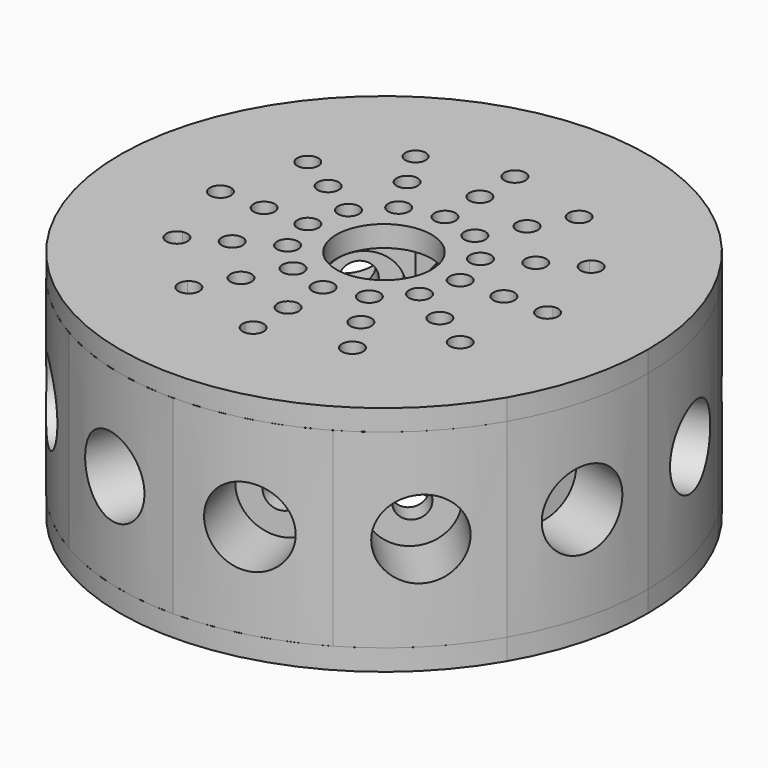
from build123d import *
from build123d import SkipClean  # not in build123d's __all__

# Parameters (mm, degrees)
F1_DEPTH  = 18
F2_R      = 3.35
F2_R_2    = 1.5
F3_DEPTH  = 2
F4_DEPTH  = 12
F6_R      = 3.7
F7_DEPTH  = 12
F8_R      = 1
F9_DEPTH  = 2
F10_R     = 1
F11_DEPTH = 2
F12_COUNT = 12
F13_R     = 1
F13_R_2   = 0.75
F13_R_3   = 4.5
F14_DEPTH = 2
F15_DEPTH = 1.5
F16_R     = 1
F16_R_2   = 1.0601015706
F16_R_3   = 4.5
F16_R_4   = 0.75
F17_DEPTH = 2
F18_DEPTH = 1.5


with BuildPart() as f1:
    # F0 (on Top) → F1 (new body)
    with BuildSketch(Plane.XY):
        with BuildLine():
            Line((7.75, 13.4233937587), (12.5, 21.6506350946))
            ThreePointArc((12.5, 21.6506350946), (6.4704761276, 24.1481456572), (0, 25))
            Line((0, 25), (0, 15.5))
            Line((0, 15.5), (7.75, 13.4233937587))
        make_face()
    extrude(amount=F1_DEPTH)

    # F2 (on face) → F3 (cut)
    with BuildSketch(Plane(origin=(3.875, 14.4616968793, 0), x_dir=(0.9659258263, -0.2588190451, 0), z_dir=(-0.2588190451, -0.9659258263, 0))):
        with Locations((0, 9)):
            Circle(F2_R)
        with Locations((0, 9)):
            Circle(F2_R_2, mode=Mode.SUBTRACT)
    extrude(amount=-F3_DEPTH, mode=Mode.SUBTRACT)

    # F4 (cut): a face of the model
    f4_faces = [f1.faces().sort_by_distance(p)[0] for p in [
        (3.875, 14.4616968793, 9),
    ]]
    extrude(f4_faces, amount=-F4_DEPTH, mode=Mode.SUBTRACT)

    # F6 (on offset) → F7 (cut)
    with BuildSketch(Plane(origin=(4.9102761804, 18.3254001845, 0), x_dir=(0.9659258263, -0.2588190451, 0), z_dir=(-0.2588190451, -0.9659258263, 0))):
        with Locations((0, 9)):
            Circle(F6_R)
    extrude(amount=-F7_DEPTH, mode=Mode.SUBTRACT)

    # F8 (on face) → F9 (cut)
    with BuildSketch(Plane.XY.offset(18)):
        with Locations((9.7439876188, 20.8650568617)):
            Circle(F8_R)
    extrude(amount=-F9_DEPTH, mode=Mode.SUBTRACT)

    # F10 (on face) → F11 (cut)
    with BuildSketch(Plane(origin=(0, 0, 0), x_dir=(1, 0, 0), z_dir=(0, 0, -1))):
        with Locations((1.9939876188, -22.941663103)):
            Circle(F10_R)
    extrude(amount=-F11_DEPTH, mode=Mode.SUBTRACT)

    # F12: F1 ×12 about axis
    f12_axis = Axis((0, 0, 0), (0, 0, 1))


with BuildPart() as f1_1:
    add(f1.part, clean=False)
    with SkipClean():  # cleaning this boolean's faces spoils the solid; the shape is the same uncleaned
        for i in range(1, F12_COUNT):
            add(f1.part.rotate(f12_axis, i * 360 / F12_COUNT), clean=False)


with BuildPart() as f14:
    # F13 (on face) → F14 (new body)
    with BuildSketch(Plane.XY.offset(18)):
        with BuildLine():
            Line((14.2894191624, 8.25), (21.6506350946, 12.5))
            ThreePointArc((21.6506350946, 12.5), (17.6776695297, 17.6776695297), (12.5, 21.6506350946))
            Line((12.5, 21.6506350946), (8.25, 14.2894191624))
            ThreePointArc((8.25, 14.2894191624), (8.6160254038, 13.9233937587), (8.75, 13.4233937587))
            ThreePointArc((8.75, 13.4233937587), (8.6738795325, 13.0407103263), (8.4571067812, 12.7162869775))
            Line((8.4571067812, 12.7162869775), (12.7162869775, 8.4571067812))
            ThreePointArc((12.7162869775, 8.4571067812), (13.5539199509, 8.7414448614), (14.2894191624, 8.25))
        make_face()
        with Locations((18.8710692429, 13.1976754842)):
            Circle(F13_R, mode=Mode.SUBTRACT)
        with BuildLine():
            ThreePointArc((21.6506350946, -12.5), (24.1481456572, -6.4704761276), (25, 0))
            ThreePointArc((25, 0), (24.1481456572, 6.4704761276), (21.6506350946, 12.5))
            Line((21.6506350946, 12.5), (14.2894191624, 8.25))
            ThreePointArc((14.2894191624, 8.25), (14.3893195849, 8.0088190451), (14.4233937587, 7.75))
            ThreePointArc((14.4233937587, 7.75), (14.216747099, 7.141238571), (13.6822128038, 6.7840741737))
            Line((13.6822128038, 6.7840741737), (15.2411809549, 0.9659258263))
            ThreePointArc((15.2411809549, 0.9659258263), (16.108761429, 0.7933533403), (16.5, 0))
            ThreePointArc((16.5, 0), (16.108761429, -0.7933533403), (15.2411809549, -0.9659258263))
            Line((15.2411809549, -0.9659258263), (13.6822128038, -6.7840741737))
            ThreePointArc((13.6822128038, -6.7840741737), (14.216747099, -7.141238571), (14.4233937587, -7.75))
            ThreePointArc((14.4233937587, -7.75), (13.806077191, -8.6738795325), (12.7162869775, -8.4571067812))
            Line((12.7162869775, -8.4571067812), (8.4571067812, -12.7162869775))
            ThreePointArc((8.4571067812, -12.7162869775), (8.6738795325, -13.0407103263), (8.75, -13.4233937587))
            ThreePointArc((8.75, -13.4233937587), (7.8805261922, -14.41483862), (6.7840741737, -13.6822128038))
            Line((6.7840741737, -13.6822128038), (0.9659258263, -15.2411809549))
            ThreePointArc((0.9659258263, -15.2411809549), (0.9914448614, -15.3694738078), (1, -15.5))
            ThreePointArc((1, -15.5), (-0.1305261922, -16.4914448614), (-0.9659258263, -15.2411809549))
            Line((-0.9659258263, -15.2411809549), (-6.7840741737, -13.6822128038))
            ThreePointArc((-6.7840741737, -13.6822128038), (-8.25, -14.2894191624), (-8.4571067812, -12.7162869775))
            Line((-8.4571067812, -12.7162869775), (-12.7162869775, -8.4571067812))
            ThreePointArc((-12.7162869775, -8.4571067812), (-14.2894191624, -8.25), (-13.6822128038, -6.7840741737))
            Line((-13.6822128038, -6.7840741737), (-15.2411809549, -0.9659258263))
            ThreePointArc((-15.2411809549, -0.9659258263), (-16.5, 0), (-15.2411809549, 0.9659258263))
            Line((-15.2411809549, 0.9659258263), (-13.6822128038, 6.7840741737))
            ThreePointArc((-13.6822128038, 6.7840741737), (-14.2894191624, 8.25), (-12.7162869775, 8.4571067812))
            Line((-12.7162869775, 8.4571067812), (-8.4328611299, 12.7405326287))
            ThreePointArc((-8.4328611299, 12.7405326287), (-8.2328557356, 14.2597244254), (-6.8171943493, 13.6733382795))
            Line((-6.8171943493, 13.6733382795), (-0.9659258263, 15.2411809549))
            ThreePointArc((-0.9659258263, 15.2411809549), (-0.1305261922, 16.4914448614), (1, 15.5))
            ThreePointArc((1, 15.5), (0.9914448614, 15.3694738078), (0.9659258263, 15.2411809549))
            Line((0.9659258263, 15.2411809549), (6.7840741737, 13.6822128038))
            ThreePointArc((6.7840741737, 13.6822128038), (7.3673165676, 14.3472732912), (8.25, 14.2894191624))
            Line((8.25, 14.2894191624), (12.5, 21.6506350946))
            ThreePointArc((12.5, 21.6506350946), (-24.1481456572, -6.4704761276), (21.6506350946, -12.5))
        make_face()
        with Locations((-18.8710692429, -13.1976754842)):
            Circle(F13_R, mode=Mode.SUBTRACT)
        with Locations((-9.7439876188, -20.8650568617)):
            Circle(F13_R, mode=Mode.SUBTRACT)
        with Locations((-22.941663103, -1.9939876188)):
            Circle(F13_R, mode=Mode.SUBTRACT)
        with Locations((1.9939876188, -22.941663103)):
            Circle(F13_R, mode=Mode.SUBTRACT)
        with Locations((13.1976754842, -18.8710692429)):
            Circle(F13_R, mode=Mode.SUBTRACT)
        with Locations((20.8650568617, -9.7439876188)):
            Circle(F13_R, mode=Mode.SUBTRACT)
        with Locations((-20.8650568617, 9.7439876188)):
            Circle(F13_R, mode=Mode.SUBTRACT)
        with Locations((-13.1976754842, 18.8710692429)):
            Circle(F13_R, mode=Mode.SUBTRACT)
        with Locations((-1.9939876188, 22.941663103)):
            Circle(F13_R, mode=Mode.SUBTRACT)
        with Locations((22.941663103, 1.9939876188)):
            Circle(F13_R, mode=Mode.SUBTRACT)
        with Locations((9.7439876188, 20.8650568617)):
            Circle(F13_R, mode=Mode.SUBTRACT)
        with Locations((-20.8650568617, 9.7439876188)):
            Circle(F13_R)
        with Locations((-20.8650568617, 9.7439876188)):
            Circle(F13_R_2, mode=Mode.SUBTRACT)
        with Locations((-22.941663103, -1.9939876188)):
            Circle(F13_R)
        with Locations((-22.941663103, -1.9939876188)):
            Circle(F13_R_2, mode=Mode.SUBTRACT)
        with BuildLine():
            ThreePointArc((13.6822128038, 6.7840741737), (12.5573683549, 7.25), (12.7162869775, 8.4571067812))
            Line((12.7162869775, 8.4571067812), (8.4571067812, 12.7162869775))
            ThreePointArc((8.4571067812, 12.7162869775), (7.25, 12.5573683549), (6.7840741737, 13.6822128038))
            Line((6.7840741737, 13.6822128038), (0.9659258263, 15.2411809549))
            ThreePointArc((0.9659258263, 15.2411809549), (0, 14.5), (-0.9659258263, 15.2411809549))
            Line((-0.9659258263, 15.2411809549), (-6.8171943493, 13.6733382795))
            ThreePointArc((-6.8171943493, 13.6733382795), (-6.7925503244, 13.5494443998), (-6.7842885289, 13.4233937587))
            ThreePointArc((-6.7842885289, 13.4233937587), (-7.3804382195, 12.5311926962), (-8.4328611299, 12.7405326287))
            Line((-8.4328611299, 12.7405326287), (-12.7162869775, 8.4571067812))
            ThreePointArc((-12.7162869775, 8.4571067812), (-12.4995142261, 8.1326834324), (-12.4233937587, 7.75))
            ThreePointArc((-12.4233937587, 7.75), (-12.8146323297, 6.9566466597), (-13.6822128038, 6.7840741737))
            Line((-13.6822128038, 6.7840741737), (-15.2411809549, 0.9659258263))
            ThreePointArc((-15.2411809549, 0.9659258263), (-14.7066466597, 0.608761429), (-14.5, 0))
            ThreePointArc((-14.5, 0), (-14.7066466597, -0.608761429), (-15.2411809549, -0.9659258263))
            Line((-15.2411809549, -0.9659258263), (-13.6822128038, -6.7840741737))
            ThreePointArc((-13.6822128038, -6.7840741737), (-12.8146323297, -6.9566466597), (-12.4233937587, -7.75))
            ThreePointArc((-12.4233937587, -7.75), (-12.4995142261, -8.1326834324), (-12.7162869775, -8.4571067812))
            Line((-12.7162869775, -8.4571067812), (-8.4571067812, -12.7162869775))
            ThreePointArc((-8.4571067812, -12.7162869775), (-7.3673165676, -12.4995142261), (-6.75, -13.4233937587))
            ThreePointArc((-6.75, -13.4233937587), (-6.7585551386, -13.5539199509), (-6.7840741737, -13.6822128038))
            Line((-6.7840741737, -13.6822128038), (-0.9659258263, -15.2411809549))
            ThreePointArc((-0.9659258263, -15.2411809549), (0, -14.5), (0.9659258263, -15.2411809549))
            Line((0.9659258263, -15.2411809549), (6.7840741737, -13.6822128038))
            ThreePointArc((6.7840741737, -13.6822128038), (7.25, -12.5573683549), (8.4571067812, -12.7162869775))
            Line((8.4571067812, -12.7162869775), (12.7162869775, -8.4571067812))
            ThreePointArc((12.7162869775, -8.4571067812), (12.5573683549, -7.25), (13.6822128038, -6.7840741737))
            Line((13.6822128038, -6.7840741737), (15.2411809549, -0.9659258263))
            ThreePointArc((15.2411809549, -0.9659258263), (14.5, 0), (15.2411809549, 0.9659258263))
            Line((15.2411809549, 0.9659258263), (13.6822128038, 6.7840741737))
        make_face()
        with Locations((-5.6794476392, -9.83709187)):
            Circle(F13_R, mode=Mode.SUBTRACT)
        with Locations((-3.6088952784, -6.2507899813)):
            Circle(F13_R, mode=Mode.SUBTRACT)
        with Locations((-9.83709187, -5.6794476392)):
            Circle(F13_R, mode=Mode.SUBTRACT)
        with Locations((-6.2507899813, -3.6088952784)):
            Circle(F13_R, mode=Mode.SUBTRACT)
        with Locations((0, -11.3588952784)):
            Circle(F13_R, mode=Mode.SUBTRACT)
        with Locations((5.6794476392, -9.83709187)):
            Circle(F13_R, mode=Mode.SUBTRACT)
        with Locations((0, -7.2177905567)):
            Circle(F13_R, mode=Mode.SUBTRACT)
        with Locations((3.6088952784, -6.2507899813)):
            Circle(F13_R, mode=Mode.SUBTRACT)
        with Locations((6.2507899813, -3.6088952784)):
            Circle(F13_R, mode=Mode.SUBTRACT)
        with Locations((9.83709187, -5.6794476392)):
            Circle(F13_R, mode=Mode.SUBTRACT)
        with Locations((-11.3588952784, 0)):
            Circle(F13_R, mode=Mode.SUBTRACT)
        with Locations((-7.2177905567, 0)):
            Circle(F13_R, mode=Mode.SUBTRACT)
        with Locations((-9.83709187, 5.6794476392)):
            Circle(F13_R, mode=Mode.SUBTRACT)
        with Locations((-6.2507899813, 3.6088952784)):
            Circle(F13_R, mode=Mode.SUBTRACT)
        with Locations((-3.6088952784, 6.2507899813)):
            Circle(F13_R, mode=Mode.SUBTRACT)
        with Locations((-5.6794476392, 9.83709187)):
            Circle(F13_R, mode=Mode.SUBTRACT)
        Circle(F13_R_3, mode=Mode.SUBTRACT)
        with Locations((7.2177905567, 0)):
            Circle(F13_R, mode=Mode.SUBTRACT)
        with Locations((11.3588952784, 0)):
            Circle(F13_R, mode=Mode.SUBTRACT)
        with Locations((6.2507899813, 3.6088952784)):
            Circle(F13_R, mode=Mode.SUBTRACT)
        with Locations((9.83709187, 5.6794476392)):
            Circle(F13_R, mode=Mode.SUBTRACT)
        with Locations((0, 7.2177905567)):
            Circle(F13_R, mode=Mode.SUBTRACT)
        with Locations((3.6088952784, 6.2507899813)):
            Circle(F13_R, mode=Mode.SUBTRACT)
        with Locations((0, 11.3588952784)):
            Circle(F13_R, mode=Mode.SUBTRACT)
        with Locations((5.6794476392, 9.83709187)):
            Circle(F13_R, mode=Mode.SUBTRACT)
        with Locations((-18.8710692429, -13.1976754842)):
            Circle(F13_R)
        with Locations((-18.8710692429, -13.1976754842)):
            Circle(F13_R_2, mode=Mode.SUBTRACT)
        with Locations((-9.7439876188, -20.8650568617)):
            Circle(F13_R)
        with Locations((-9.7439876188, -20.8650568617)):
            Circle(F13_R_2, mode=Mode.SUBTRACT)
        with Locations((1.9939876188, -22.941663103)):
            Circle(F13_R)
        with Locations((1.9939876188, -22.941663103)):
            Circle(F13_R_2, mode=Mode.SUBTRACT)
        with Locations((13.1976754842, -18.8710692429)):
            Circle(F13_R)
        with Locations((13.1976754842, -18.8710692429)):
            Circle(F13_R_2, mode=Mode.SUBTRACT)
        with Locations((20.8650568617, -9.7439876188)):
            Circle(F13_R)
        with Locations((20.8650568617, -9.7439876188)):
            Circle(F13_R_2, mode=Mode.SUBTRACT)
        with Locations((22.941663103, 1.9939876188)):
            Circle(F13_R)
        with Locations((22.941663103, 1.9939876188)):
            Circle(F13_R_2, mode=Mode.SUBTRACT)
        with Locations((18.8710692429, 13.1976754842)):
            Circle(F13_R)
        with Locations((18.8710692429, 13.1976754842)):
            Circle(F13_R_2, mode=Mode.SUBTRACT)
        with Locations((9.7439876188, 20.8650568617)):
            Circle(F13_R)
        with Locations((9.7439876188, 20.8650568617)):
            Circle(F13_R_2, mode=Mode.SUBTRACT)
        with Locations((-1.9939876188, 22.941663103)):
            Circle(F13_R)
        with Locations((-1.9939876188, 22.941663103)):
            Circle(F13_R_2, mode=Mode.SUBTRACT)
        with Locations((-13.1976754842, 18.8710692429)):
            Circle(F13_R)
        with Locations((-13.1976754842, 18.8710692429)):
            Circle(F13_R_2, mode=Mode.SUBTRACT)
        with Locations((-22.941663103, -1.9939876188)):
            Circle(F13_R_2)
        with Locations((-20.8650568617, 9.7439876188)):
            Circle(F13_R_2)
        with Locations((-18.8710692429, -13.1976754842)):
            Circle(F13_R_2)
        with Locations((20.8650568617, -9.7439876188)):
            Circle(F13_R_2)
        with Locations((22.941663103, 1.9939876188)):
            Circle(F13_R_2)
        with Locations((18.8710692429, 13.1976754842)):
            Circle(F13_R_2)
        with Locations((-9.7439876188, -20.8650568617)):
            Circle(F13_R_2)
        with Locations((1.9939876188, -22.941663103)):
            Circle(F13_R_2)
        with Locations((13.1976754842, -18.8710692429)):
            Circle(F13_R_2)
        with Locations((-1.9939876188, 22.941663103)):
            Circle(F13_R_2)
        with Locations((9.7439876188, 20.8650568617)):
            Circle(F13_R_2)
        with Locations((-13.1976754842, 18.8710692429)):
            Circle(F13_R_2)
    extrude(amount=F14_DEPTH)

    # F13 (on face) → F15 (join)
    with BuildSketch(Plane.XY.offset(18)):
        with Locations((-13.1976754842, 18.8710692429)):
            Circle(F13_R_2)
        with Locations((-1.9939876188, 22.941663103)):
            Circle(F13_R_2)
        with Locations((9.7439876188, 20.8650568617)):
            Circle(F13_R_2)
        with Locations((-20.8650568617, 9.7439876188)):
            Circle(F13_R_2)
        with Locations((-22.941663103, -1.9939876188)):
            Circle(F13_R_2)
        with Locations((-18.8710692429, -13.1976754842)):
            Circle(F13_R_2)
        with Locations((-9.7439876188, -20.8650568617)):
            Circle(F13_R_2)
        with Locations((1.9939876188, -22.941663103)):
            Circle(F13_R_2)
        with Locations((13.1976754842, -18.8710692429)):
            Circle(F13_R_2)
        with Locations((20.8650568617, -9.7439876188)):
            Circle(F13_R_2)
        with Locations((22.941663103, 1.9939876188)):
            Circle(F13_R_2)
        with Locations((18.8710692429, 13.1976754842)):
            Circle(F13_R_2)
    extrude(amount=-F15_DEPTH)


with BuildPart() as f17:
    # F16 (on face) → F17 (new body)
    with BuildSketch(Plane(origin=(0, 0, 0), x_dir=(1, 0, 0), z_dir=(0, 0, -1))):
        with BuildLine():
            ThreePointArc((12.5, -21.6506350946), (17.6776695297, -17.6776695297), (21.6506350946, -12.5))
            Line((21.6506350946, -12.5), (14.2894191624, -8.25))
            ThreePointArc((14.2894191624, -8.25), (13.5539199509, -8.7414448614), (12.7162869775, -8.4571067812))
            Line((12.7162869775, -8.4571067812), (8.4571067812, -12.7162869775))
            ThreePointArc((8.4571067812, -12.7162869775), (8.6738795325, -13.0407103263), (8.75, -13.4233937587))
            ThreePointArc((8.75, -13.4233937587), (8.6160254038, -13.9233937587), (8.25, -14.2894191624))
            Line((8.25, -14.2894191624), (12.5, -21.6506350946))
        make_face()
        with Locations((13.1976754842, -18.8710692429)):
            Circle(F16_R, mode=Mode.SUBTRACT)
        with BuildLine():
            ThreePointArc((21.6506350946, -12.5), (24.1481456572, -6.4704761276), (25, 0))
            ThreePointArc((25, 0), (24.1481456572, 6.4704761276), (21.6506350946, 12.5))
            ThreePointArc((21.6506350946, 12.5), (-24.1481456572, 6.4704761276), (12.5, -21.6506350946))
            Line((12.5, -21.6506350946), (8.25, -14.2894191624))
            ThreePointArc((8.25, -14.2894191624), (7.3673165676, -14.3472732912), (6.7840741737, -13.6822128038))
            Line((6.7840741737, -13.6822128038), (0.9659258263, -15.2411809549))
            ThreePointArc((0.9659258263, -15.2411809549), (0.9914448614, -15.3694738078), (1, -15.5))
            ThreePointArc((1, -15.5), (-0.1305261922, -16.4914448614), (-0.9659258263, -15.2411809549))
            Line((-0.9659258263, -15.2411809549), (-6.7840741737, -13.6822128038))
            ThreePointArc((-6.7840741737, -13.6822128038), (-8.25, -14.2894191624), (-8.4571067812, -12.7162869775))
            Line((-8.4571067812, -12.7162869775), (-12.7162869775, -8.4571067812))
            ThreePointArc((-12.7162869775, -8.4571067812), (-14.2894191624, -8.25), (-13.6822128038, -6.7840741737))
            Line((-13.6822128038, -6.7840741737), (-15.2411809549, -0.9659258263))
            ThreePointArc((-15.2411809549, -0.9659258263), (-16.5, 0), (-15.2411809549, 0.9659258263))
            Line((-15.2411809549, 0.9659258263), (-13.6822128038, 6.7840741737))
            ThreePointArc((-13.6822128038, 6.7840741737), (-14.2894191624, 8.25), (-12.7162869775, 8.4571067812))
            Line((-12.7162869775, 8.4571067812), (-8.4571067812, 12.7162869775))
            ThreePointArc((-8.4571067812, 12.7162869775), (-8.25, 14.2894191624), (-6.7840741737, 13.6822128038))
            Line((-6.7840741737, 13.6822128038), (-0.9659258263, 15.2411809549))
            ThreePointArc((-0.9659258263, 15.2411809549), (-0.1305261922, 16.4914448614), (1, 15.5))
            ThreePointArc((1, 15.5), (0.9914448614, 15.3694738078), (0.9659258263, 15.2411809549))
            Line((0.9659258263, 15.2411809549), (6.7840741737, 13.6822128038))
            ThreePointArc((6.7840741737, 13.6822128038), (7.8805261922, 14.41483862), (8.75, 13.4233937587))
            ThreePointArc((8.75, 13.4233937587), (8.6738795325, 13.0407103263), (8.4571067812, 12.7162869775))
            Line((8.4571067812, 12.7162869775), (12.7162869775, 8.4571067812))
            ThreePointArc((12.7162869775, 8.4571067812), (13.806077191, 8.6738795325), (14.4233937587, 7.75))
            ThreePointArc((14.4233937587, 7.75), (14.216747099, 7.141238571), (13.6822128038, 6.7840741737))
            Line((13.6822128038, 6.7840741737), (15.2411809549, 0.9659258263))
            ThreePointArc((15.2411809549, 0.9659258263), (16.108761429, 0.7933533403), (16.5, 0))
            ThreePointArc((16.5, 0), (16.108761429, -0.7933533403), (15.2411809549, -0.9659258263))
            Line((15.2411809549, -0.9659258263), (13.6822128038, -6.7840741737))
            ThreePointArc((13.6822128038, -6.7840741737), (14.216747099, -7.141238571), (14.4233937587, -7.75))
            ThreePointArc((14.4233937587, -7.75), (14.3893195849, -8.0088190451), (14.2894191624, -8.25))
            Line((14.2894191624, -8.25), (21.6506350946, -12.5))
        make_face()
        with Locations((-18.8710692429, -13.1976754842)):
            Circle(F16_R, mode=Mode.SUBTRACT)
        with Locations((-9.7439876188, -20.8650568617)):
            Circle(F16_R, mode=Mode.SUBTRACT)
        with Locations((-22.941663103, -1.9939876188)):
            Circle(F16_R, mode=Mode.SUBTRACT)
        with Locations((1.9939876188, -22.941663103)):
            Circle(F16_R, mode=Mode.SUBTRACT)
        with Locations((20.8650568617, -9.7439876188)):
            Circle(F16_R, mode=Mode.SUBTRACT)
        with Locations((-20.8650568617, 9.7439876188)):
            Circle(F16_R, mode=Mode.SUBTRACT)
        with Locations((-13.1976754842, 18.8710692429)):
            Circle(F16_R, mode=Mode.SUBTRACT)
        with Locations((-1.9939876188, 22.941663103)):
            Circle(F16_R, mode=Mode.SUBTRACT)
        with Locations((22.941663103, 1.9939876188)):
            Circle(F16_R, mode=Mode.SUBTRACT)
        with Locations((9.7439876188, 20.8650568617)):
            Circle(F16_R, mode=Mode.SUBTRACT)
        with Locations((18.8710692429, 13.1976754842)):
            Circle(F16_R, mode=Mode.SUBTRACT)
        with BuildLine():
            Line((8.4571067812, -12.7162869775), (12.7162869775, -8.4571067812))
            ThreePointArc((12.7162869775, -8.4571067812), (12.5573683549, -7.25), (13.6822128038, -6.7840741737))
            Line((13.6822128038, -6.7840741737), (15.2411809549, -0.9659258263))
            ThreePointArc((15.2411809549, -0.9659258263), (14.5, 0), (15.2411809549, 0.9659258263))
            Line((15.2411809549, 0.9659258263), (13.6822128038, 6.7840741737))
            ThreePointArc((13.6822128038, 6.7840741737), (12.5573683549, 7.25), (12.7162869775, 8.4571067812))
            Line((12.7162869775, 8.4571067812), (8.4571067812, 12.7162869775))
            ThreePointArc((8.4571067812, 12.7162869775), (7.25, 12.5573683549), (6.7840741737, 13.6822128038))
            Line((6.7840741737, 13.6822128038), (0.9659258263, 15.2411809549))
            ThreePointArc((0.9659258263, 15.2411809549), (0, 14.5), (-0.9659258263, 15.2411809549))
            Line((-0.9659258263, 15.2411809549), (-6.7840741737, 13.6822128038))
            ThreePointArc((-6.7840741737, 13.6822128038), (-6.7585551386, 13.5539199509), (-6.75, 13.4233937587))
            ThreePointArc((-6.75, 13.4233937587), (-7.3673165676, 12.4995142261), (-8.4571067812, 12.7162869775))
            Line((-8.4571067812, 12.7162869775), (-12.7162869775, 8.4571067812))
            ThreePointArc((-12.7162869775, 8.4571067812), (-12.4995142261, 8.1326834324), (-12.4233937587, 7.75))
            ThreePointArc((-12.4233937587, 7.75), (-12.8146323297, 6.9566466597), (-13.6822128038, 6.7840741737))
            Line((-13.6822128038, 6.7840741737), (-15.2411809549, 0.9659258263))
            ThreePointArc((-15.2411809549, 0.9659258263), (-14.7066466597, 0.608761429), (-14.5, 0))
            ThreePointArc((-14.5, 0), (-14.7066466597, -0.608761429), (-15.2411809549, -0.9659258263))
            Line((-15.2411809549, -0.9659258263), (-13.6822128038, -6.7840741737))
            ThreePointArc((-13.6822128038, -6.7840741737), (-12.8146323297, -6.9566466597), (-12.4233937587, -7.75))
            ThreePointArc((-12.4233937587, -7.75), (-12.4995142261, -8.1326834324), (-12.7162869775, -8.4571067812))
            Line((-12.7162869775, -8.4571067812), (-8.4571067812, -12.7162869775))
            ThreePointArc((-8.4571067812, -12.7162869775), (-7.3673165676, -12.4995142261), (-6.75, -13.4233937587))
            ThreePointArc((-6.75, -13.4233937587), (-6.7585551386, -13.5539199509), (-6.7840741737, -13.6822128038))
            Line((-6.7840741737, -13.6822128038), (-0.9659258263, -15.2411809549))
            ThreePointArc((-0.9659258263, -15.2411809549), (0, -14.5), (0.9659258263, -15.2411809549))
            Line((0.9659258263, -15.2411809549), (6.7840741737, -13.6822128038))
            ThreePointArc((6.7840741737, -13.6822128038), (7.25, -12.5573683549), (8.4571067812, -12.7162869775))
        make_face()
        with Locations((-5.6794476392, -9.83709187)):
            Circle(F16_R, mode=Mode.SUBTRACT)
        with Locations((-3.6088952784, -6.2507899813)):
            Circle(F16_R, mode=Mode.SUBTRACT)
        with Locations((-9.83709187, -5.6794476392)):
            Circle(F16_R, mode=Mode.SUBTRACT)
        with Locations((-6.2507899813, -3.6088952784)):
            Circle(F16_R, mode=Mode.SUBTRACT)
        with Locations((0, -11.3588952784)):
            Circle(F16_R_2, mode=Mode.SUBTRACT)
        with Locations((5.6794476392, -9.83709187)):
            Circle(F16_R, mode=Mode.SUBTRACT)
        with Locations((0, -7.2177905567)):
            Circle(F16_R, mode=Mode.SUBTRACT)
        with Locations((3.6088952784, -6.2507899813)):
            Circle(F16_R, mode=Mode.SUBTRACT)
        with Locations((6.2507899813, -3.6088952784)):
            Circle(F16_R, mode=Mode.SUBTRACT)
        with Locations((9.83709187, -5.6794476392)):
            Circle(F16_R, mode=Mode.SUBTRACT)
        with Locations((-11.3588952784, 0)):
            Circle(F16_R, mode=Mode.SUBTRACT)
        with Locations((-7.2177905567, 0)):
            Circle(F16_R, mode=Mode.SUBTRACT)
        with Locations((-9.83709187, 5.6794476392)):
            Circle(F16_R, mode=Mode.SUBTRACT)
        with Locations((-6.2507899813, 3.6088952784)):
            Circle(F16_R, mode=Mode.SUBTRACT)
        with Locations((-3.6088952784, 6.2507899813)):
            Circle(F16_R, mode=Mode.SUBTRACT)
        with Locations((-5.6794476392, 9.83709187)):
            Circle(F16_R, mode=Mode.SUBTRACT)
        Circle(F16_R_3, mode=Mode.SUBTRACT)
        with Locations((7.2177905567, 0)):
            Circle(F16_R, mode=Mode.SUBTRACT)
        with Locations((11.3588952784, 0)):
            Circle(F16_R, mode=Mode.SUBTRACT)
        with Locations((6.2507899813, 3.6088952784)):
            Circle(F16_R, mode=Mode.SUBTRACT)
        with Locations((9.83709187, 5.6794476392)):
            Circle(F16_R, mode=Mode.SUBTRACT)
        with Locations((0, 7.2177905567)):
            Circle(F16_R, mode=Mode.SUBTRACT)
        with Locations((3.6088952784, 6.2507899813)):
            Circle(F16_R, mode=Mode.SUBTRACT)
        with Locations((0, 11.3588952784)):
            Circle(F16_R, mode=Mode.SUBTRACT)
        with Locations((5.6794476392, 9.83709187)):
            Circle(F16_R, mode=Mode.SUBTRACT)
        with Locations((-18.8710692429, -13.1976754842)):
            Circle(F16_R)
        with Locations((-18.8710692429, -13.1976754842)):
            Circle(F16_R_4, mode=Mode.SUBTRACT)
        with Locations((-9.7439876188, -20.8650568617)):
            Circle(F16_R)
        with Locations((-9.7439876188, -20.8650568617)):
            Circle(F16_R_4, mode=Mode.SUBTRACT)
        with Locations((1.9939876188, -22.941663103)):
            Circle(F16_R)
        with Locations((1.9939876188, -22.941663103)):
            Circle(F16_R_4, mode=Mode.SUBTRACT)
        with Locations((13.1976754842, -18.8710692429)):
            Circle(F16_R)
        with Locations((13.1976754842, -18.8710692429)):
            Circle(F16_R_4, mode=Mode.SUBTRACT)
        with Locations((20.8650568617, -9.7439876188)):
            Circle(F16_R)
        with Locations((20.8650568617, -9.7439876188)):
            Circle(F16_R_4, mode=Mode.SUBTRACT)
        with Locations((22.941663103, 1.9939876188)):
            Circle(F16_R)
        with Locations((22.941663103, 1.9939876188)):
            Circle(F16_R_4, mode=Mode.SUBTRACT)
        with Locations((18.8710692429, 13.1976754842)):
            Circle(F16_R)
        with Locations((18.8710692429, 13.1976754842)):
            Circle(F16_R_4, mode=Mode.SUBTRACT)
        with Locations((9.7439876188, 20.8650568617)):
            Circle(F16_R)
        with Locations((9.7439876188, 20.8650568617)):
            Circle(F16_R_4, mode=Mode.SUBTRACT)
        with Locations((-1.9939876188, 22.941663103)):
            Circle(F16_R)
        with Locations((-1.9939876188, 22.941663103)):
            Circle(F16_R_4, mode=Mode.SUBTRACT)
        with Locations((-13.1976754842, 18.8710692429)):
            Circle(F16_R)
        with Locations((-13.1976754842, 18.8710692429)):
            Circle(F16_R_4, mode=Mode.SUBTRACT)
        with Locations((-20.8650568617, 9.7439876188)):
            Circle(F16_R)
        with Locations((-20.8650568617, 9.7439876188)):
            Circle(F16_R_4, mode=Mode.SUBTRACT)
        with Locations((-22.941663103, -1.9939876188)):
            Circle(F16_R)
        with Locations((-22.941663103, -1.9939876188)):
            Circle(F16_R_4, mode=Mode.SUBTRACT)
        with Locations((-9.7439876188, -20.8650568617)):
            Circle(F16_R_4)
        with Locations((1.9939876188, -22.941663103)):
            Circle(F16_R_4)
        with Locations((13.1976754842, -18.8710692429)):
            Circle(F16_R_4)
        with Locations((20.8650568617, -9.7439876188)):
            Circle(F16_R_4)
        with Locations((22.941663103, 1.9939876188)):
            Circle(F16_R_4)
        with Locations((-18.8710692429, -13.1976754842)):
            Circle(F16_R_4)
        with Locations((-22.941663103, -1.9939876188)):
            Circle(F16_R_4)
        with Locations((18.8710692429, 13.1976754842)):
            Circle(F16_R_4)
        with Locations((-20.8650568617, 9.7439876188)):
            Circle(F16_R_4)
        with Locations((-13.1976754842, 18.8710692429)):
            Circle(F16_R_4)
        with Locations((-1.9939876188, 22.941663103)):
            Circle(F16_R_4)
        with Locations((9.7439876188, 20.8650568617)):
            Circle(F16_R_4)
    extrude(amount=F17_DEPTH)

    # F16 (on face) → F18 (join)
    with BuildSketch(Plane(origin=(0, 0, 0), x_dir=(1, 0, 0), z_dir=(0, 0, -1))):
        with Locations((-18.8710692429, -13.1976754842)):
            Circle(F16_R_4)
        with Locations((-22.941663103, -1.9939876188)):
            Circle(F16_R_4)
        with Locations((-9.7439876188, -20.8650568617)):
            Circle(F16_R_4)
        with Locations((1.9939876188, -22.941663103)):
            Circle(F16_R_4)
        with Locations((13.1976754842, -18.8710692429)):
            Circle(F16_R_4)
        with Locations((20.8650568617, -9.7439876188)):
            Circle(F16_R_4)
        with Locations((22.941663103, 1.9939876188)):
            Circle(F16_R_4)
        with Locations((18.8710692429, 13.1976754842)):
            Circle(F16_R_4)
        with Locations((9.7439876188, 20.8650568617)):
            Circle(F16_R_4)
        with Locations((-1.9939876188, 22.941663103)):
            Circle(F16_R_4)
        with Locations((-13.1976754842, 18.8710692429)):
            Circle(F16_R_4)
        with Locations((-20.8650568617, 9.7439876188)):
            Circle(F16_R_4)
    extrude(amount=-F18_DEPTH)


solid = Compound([f1_1.part, f14.part, f17.part])
